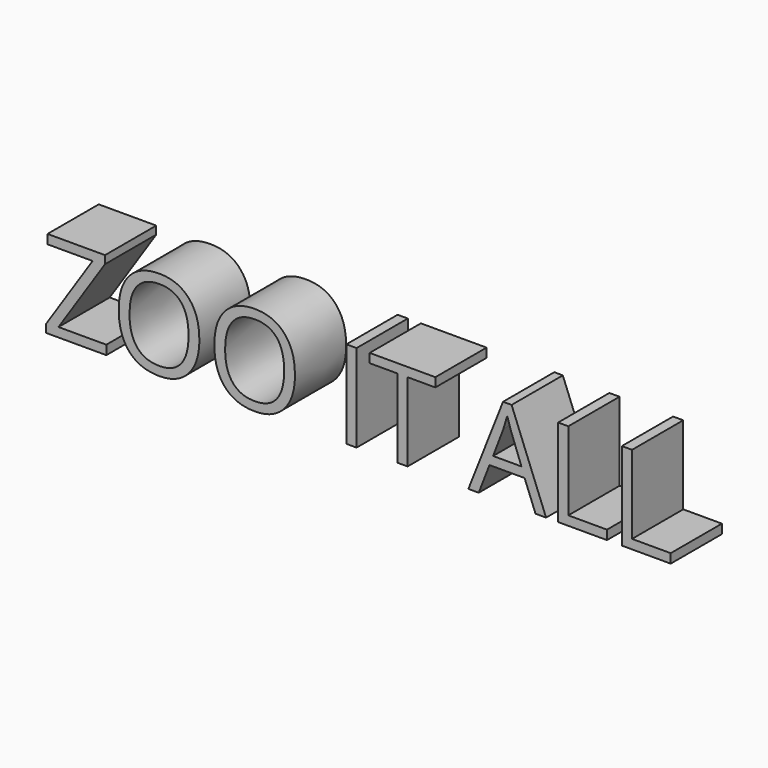
from build123d import *

# Parameters (mm, degrees)
F0_TEXT_SIZE = 48.7050041556
F1_DEPTH     = 25.4


# Not quite as in the source:
# - Text() gives the source's letters only with a copy of the font that has no kerning and outlines rounded to 1/6400 em; it was checked with that copy


with BuildPart() as f1:
    # F0 (on Front) → F1 (new body)
    with BuildSketch(Plane.XZ):
        with Locations((-112.1384678409, -26.4905262738)):
            Text('ZOO IT ALL', F0_TEXT_SIZE, font='Open Sans', text_align=(TextAlign.LEFT, TextAlign.BOTTOM))
    extrude(amount=F1_DEPTH)


solid = f1.part
